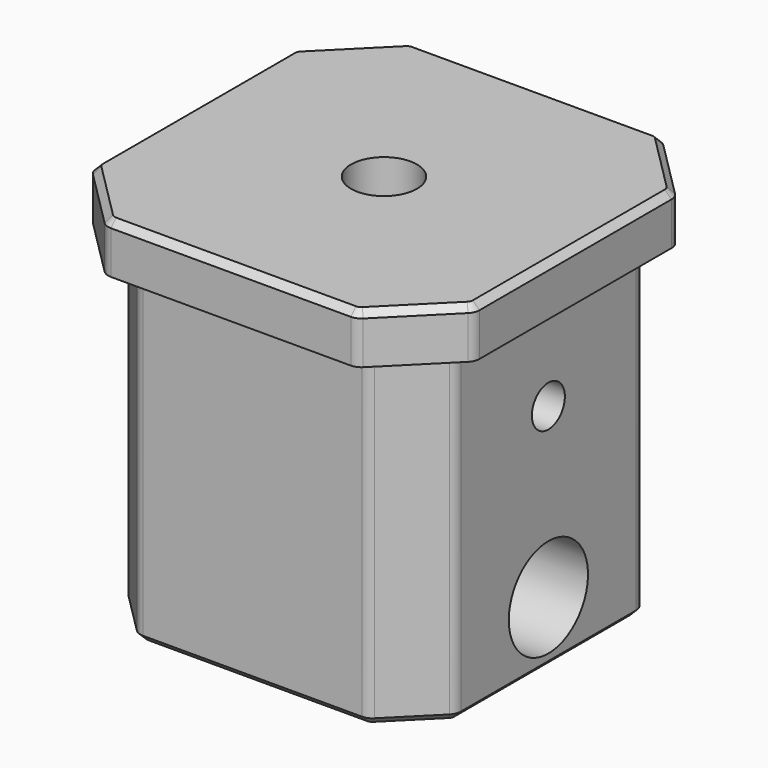
from build123d import *

# Parameters (mm, degrees)
F0_W     = 63.246
F0_H     = 63.246
F1_DEPTH = 63.5
F2_SIZE  = 9.525
F3_W     = 73.66
F3_H     = 73.66
F4_DEPTH = 9.525
F5_SIZE  = 12.7
F6_R     = 2.54
F7_SIZE  = 1.27
F8_R     = 9.525
F9_DEPTH = 68.454
F11_D    = 12.7
F13_D    = 7.9375


# Not quite as in the source:
# - a length typed as a fraction of an inch, garbled in the dataset ("3 / 203.2 mm" for 3/8 in), is restored


with BuildPart() as f1:
    # F0 (on Top) → F1 (new body)
    with BuildSketch(Plane.XY):
        Rectangle(F0_W, F0_H)
    extrude(amount=-F1_DEPTH)

    # F2
    f2_edges = [f1.edges().sort_by_distance(p)[0] for p in [
        (-31.623, -31.623, -31.75),
        (-31.623, 31.623, -31.75),
        (31.623, -31.623, -31.75),
        (31.623, 31.623, -31.75),
    ]]
    chamfer(f2_edges, length=F2_SIZE)

    # F3 (on face) → F4 (join)
    with BuildSketch(Plane.XY):
        Rectangle(F3_W, F3_H)
    extrude(amount=F4_DEPTH)

    # F5
    f5_edges = [f1.edges().sort_by_distance(p)[0] for p in [
        (36.83, -36.83, 4.7625),
        (-36.83, -36.83, 4.7625),
        (36.83, 36.83, 4.7625),
        (-36.83, 36.83, 4.7625),
    ]]
    chamfer(f5_edges, length=F5_SIZE)

    # F6
    f6_edges = [f1.edges().sort_by_distance(p)[0] for p in [
        (-24.13, -36.83, 4.7625),
        (24.13, -36.83, 4.7625),
        (36.83, -24.13, 4.7625),
        (-36.83, -24.13, 4.7625),
        (36.83, 24.13, 4.7625),
        (24.13, 36.83, 4.7625),
        (-24.13, 36.83, 4.7625),
        (-36.83, 24.13, 4.7625),
        (-22.098, 31.623, -31.75),
        (-31.623, 22.098, -31.75),
        (22.098, 31.623, -31.75),
        (31.623, 22.098, -31.75),
        (-31.623, -22.098, -31.75),
        (-22.098, -31.623, -31.75),
        (31.623, -22.098, -31.75),
        (22.098, -31.623, -31.75),
    ]]
    fillet(f6_edges, radius=F6_R)

    # F7
    f7_edges = [f1.edges().sort_by_distance(p)[0] for p in [
        (-30.48, 30.48, 9.525),
        (-31.623, 0, -63.5),
    ]]
    chamfer(f7_edges, length=F7_SIZE)

    # F8 (on face) → F9 (cut, through all)
    with BuildSketch(Plane(origin=(-31.623, 0, 0), x_dir=(0, -1, 0), z_dir=(-1, 0, 0))):
        with Locations((0, -51.435)):
            Circle(F8_R)
    extrude(amount=-F9_DEPTH, mode=Mode.SUBTRACT)

    # F11 (through all)
    with Locations(Plane.XY.offset(9.525)):
        with Locations((0, 0)):
            Hole(F11_D / 2)

    # F13 (through all)
    with Locations(Plane.YZ.offset(31.623)):
        with Locations((0, -19.05)):
            Hole(F13_D / 2)


solid = f1.part
